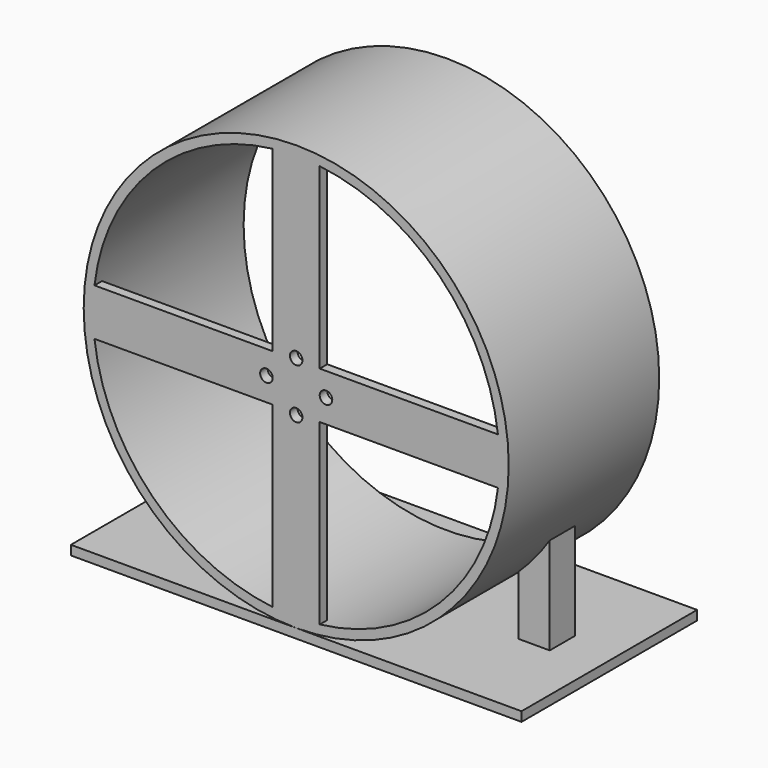
from build123d import *

# Parameters (mm, degrees)
F0_R        = 67.77
F1_DEPTH    = 60
F2_T        = -3
F4_W        = 143.71
F4_H        = 70
F5_DEPTH    = 3
F6_W        = 10
F6_H        = 10
F7_DEPTH    = 35
F8_T4_DEPTH = 77.0795565602
F8_S5_R     = 64.77
F8_T6_DEPTH = 41
F9_T4_DEPTH = 77.0795565602
F9_S5_R     = 64.77
F9_T6_DEPTH = 41
F10_W       = 15
F10_H       = 57.5
F10_W_2     = 57.5
F10_H_2     = 15
F11_DEPTH   = 3
F12_R       = 2
F13_DEPTH   = 3


# Not quite as in the source:
# - a fillet or chamfer that OpenCascade refuses, or shapes differently, is made with other operations: its cross-section is extruded or revolved along the edge and cut away or added


with BuildPart() as f1:
    # F0 (on Front) → F1 (new body)
    with BuildSketch(Plane.XZ):
        Circle(F0_R)
    extrude(amount=F1_DEPTH)

    # F2
    f2_openings = [f1.faces().sort_by_distance(p)[0] for p in [
        (0, -60, 0),
        (0, 0, 0),
    ]]
    offset(amount=F2_T, openings=f2_openings)

    # F6 (on face) → F7 (join)
    with BuildSketch(Plane.XY.offset(-67.77)):
        with Locations((-51.855, -25)):
            Rectangle(F6_W, F6_H)
        with Locations((51.855, -25)):
            Rectangle(F6_W, F6_H)
    extrude(amount=F7_DEPTH)

    # F8: chamfer of 10 x 13 on 1 edges, made by hand


with BuildPart() as f5:
    # F4 (on offset) → F5 (new body)
    with BuildSketch(Plane.XY.offset(-67.77)):
        with Locations((0, -25)):
            Rectangle(F4_W, F4_H)
    extrude(amount=-F5_DEPTH)


with BuildPart() as f8_tool2:
    # F8_s3 → F8_t4 (new body)
    with BuildSketch(Plane.XZ.offset(63.5397782801)):
        Polygon((-46.855, -45.77), (-56.855, -32.77), (-46.855, -32.77), align=None)
    extrude(amount=-F8_T4_DEPTH)

    # F8_s5 → F8_t6 (intersect, symmetric)
    with BuildSketch(Plane.XZ.offset(25)):
        Circle(F8_S5_R)
    extrude(amount=F8_T6_DEPTH, both=True, mode=Mode.INTERSECT)


with BuildPart() as f1_1:
    add(f1.part)

    # F8_t1: cut F8_tool2
    add(f8_tool2.part, mode=Mode.SUBTRACT)

    # F9: chamfer of 13 x 10 on 1 edges, made by hand


with BuildPart() as f9_tool2:
    # F9_s3 → F9_t4 (new body)
    with BuildSketch(Plane.XZ.offset(-13.5397782801)):
        Polygon((46.855, -45.77), (56.855, -32.77), (46.855, -32.77), align=None)
    extrude(amount=F9_T4_DEPTH)

    # F9_s5 → F9_t6 (intersect, symmetric)
    with BuildSketch(Plane.XZ.offset(25)):
        Circle(F9_S5_R)
    extrude(amount=F9_T6_DEPTH, both=True, mode=Mode.INTERSECT)


with BuildPart() as f1_2:
    add(f1_1.part)

    # F9_t1: cut F9_tool2
    add(f9_tool2.part, mode=Mode.SUBTRACT)

    # F10 (on face) → F11 (join)
    with BuildSketch(Plane.XZ.offset(60)):
        with Locations((0, 36.25)):
            Rectangle(F10_W, F10_H)
        with Locations((36.25, 0)):
            Rectangle(F10_W_2, F10_H_2)
        Rectangle(F10_W, F10_H_2)
        with Locations((-36.25, 0)):
            Rectangle(F10_W_2, F10_H_2)
        with Locations((0, -36.25)):
            Rectangle(F10_W, F10_H)
    extrude(amount=-F11_DEPTH)

    # F12 (on face) → F13 (cut)
    with BuildSketch(Plane.XZ.offset(60)):
        with Locations((0, 8)):
            Circle(F12_R)
        with Locations((9.5, 0)):
            Circle(F12_R)
        with Locations((-9.5, 0)):
            Circle(F12_R)
        with Locations((0, -8)):
            Circle(F12_R)
    extrude(amount=-F13_DEPTH, mode=Mode.SUBTRACT)


solid = Compound([f5.part, f1_2.part])
